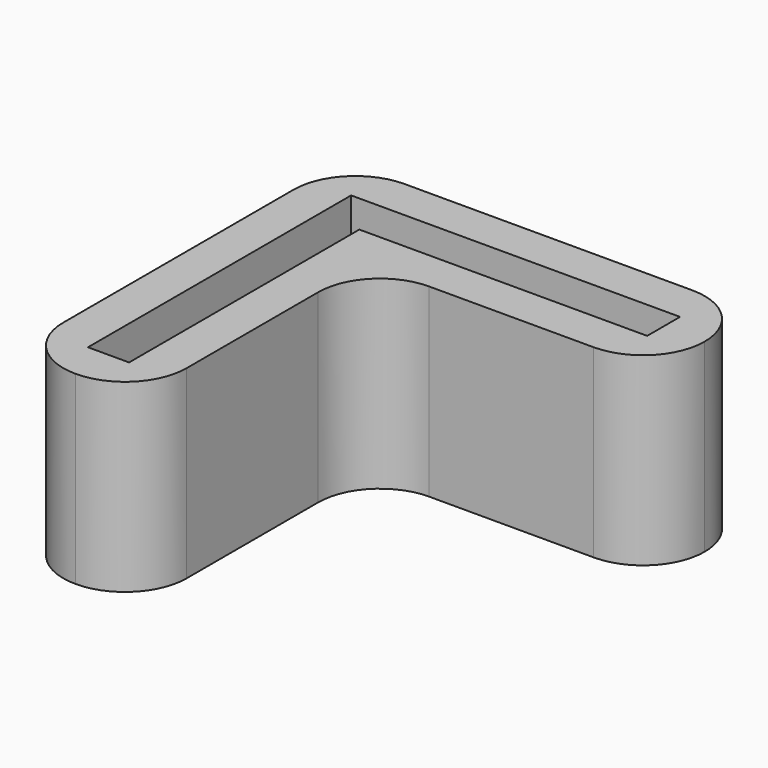
from build123d import *

# Parameters (mm, degrees)
F1_DEPTH = 2
F2_DEPTH = 7
F3_R     = 2.99999


# Not quite as in the source:
# - a fillet or chamfer is up to 0.001 mm smaller than in the source, because OpenCascade refuses the exact size


with BuildPart() as f1:
    # F0 (on Top) → F1 (new body)
    with BuildSketch(Plane.XY):
        Polygon((10.2818826017, 7.0030450644), (-7.7181173983, 7.0030450644), (-7.7181173983, -10.9969549356), (-5.7181173983, -10.9969549356), (-5.7181173983, 5.0030450644), (10.2818826017, 5.0030450644), align=None)
        Polygon((10.2818826017, 3.0030450644), (10.2818826017, 5.0030450644), (-5.7181173983, 5.0030450644), (-5.7181173983, -10.9969549356), (-3.7181173983, -10.9969549356), (-3.7181173983, 3.0030450644), align=None)
        Polygon((10.2818826017, 1.0030450644), (10.2818826017, 3.0030450644), (-3.7181173983, 3.0030450644), (-3.7181173983, -10.9969549356), (-1.7181173983, -10.9969549356), (-1.7181173983, 1.0030450644), align=None)
        Polygon((12.2818826017, 7.0030450644), (10.2818826017, 7.0030450644), (10.2818826017, 5.0030450644), (10.2818826017, 3.0030450644), (10.2818826017, 1.0030450644), (12.2818826017, 1.0030450644), align=None)
        Polygon((-5.7181173983, -10.9969549356), (-7.7181173983, -10.9969549356), (-7.7181173983, -12.9969549356), (-1.7181173983, -12.9969549356), (-1.7181173983, -10.9969549356), (-3.7181173983, -10.9969549356), align=None)
    extrude(amount=-F1_DEPTH)

    # F0 (on Top) → F2 (join)
    with BuildSketch(Plane.XY):
        Polygon((10.2818826017, 7.0030450644), (-7.7181173983, 7.0030450644), (-7.7181173983, -10.9969549356), (-5.7181173983, -10.9969549356), (-5.7181173983, 5.0030450644), (10.2818826017, 5.0030450644), align=None)
        Polygon((10.2818826017, 1.0030450644), (10.2818826017, 3.0030450644), (-3.7181173983, 3.0030450644), (-3.7181173983, -10.9969549356), (-1.7181173983, -10.9969549356), (-1.7181173983, 1.0030450644), align=None)
        Polygon((12.2818826017, 7.0030450644), (10.2818826017, 7.0030450644), (10.2818826017, 5.0030450644), (10.2818826017, 3.0030450644), (10.2818826017, 1.0030450644), (12.2818826017, 1.0030450644), align=None)
        Polygon((-5.7181173983, -10.9969549356), (-7.7181173983, -10.9969549356), (-7.7181173983, -12.9969549356), (-1.7181173983, -12.9969549356), (-1.7181173983, -10.9969549356), (-3.7181173983, -10.9969549356), align=None)
    extrude(amount=F2_DEPTH)

    # F3 (radius 3 in the source; OpenCascade refuses exactly that, so slightly less here)
    f3_edges = [f1.edges().sort_by_distance(p)[0] for p in [
        (-1.718117, 1.003045, 2.5),
        (-7.718117, 7.003045, 2.5),
        (-7.718117, -12.996955, 2.5),
        (-1.718117, -12.996955, 2.5),
        (12.281883, 1.003045, 2.5),
        (12.281883, 7.003045, 2.5),
    ]]
    fillet(f3_edges, radius=F3_R)


solid = f1.part
